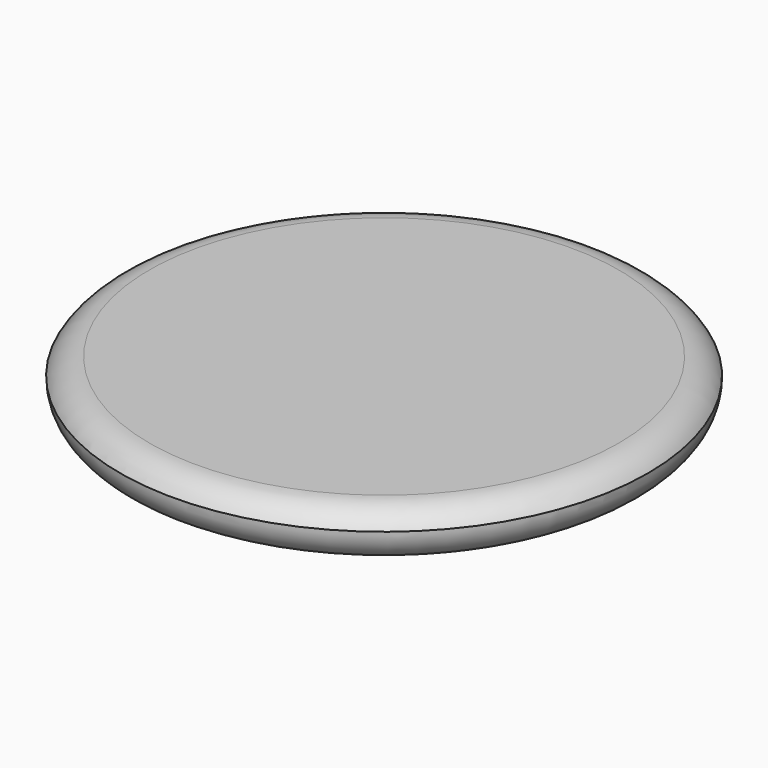
from build123d import *

# Parameters (mm, degrees)
F0_R     = 15.6
F0_R_2   = 5.6
F0_R_3   = 3.9
F1_DEPTH = 3
F2_DEPTH = 4
F3_DEPTH = 8
F4_R     = 2


# Not quite as in the source:
# - a fillet or chamfer that OpenCascade refuses, or shapes differently, is made with other operations: its cross-section is extruded or revolved along the edge and cut away or added


with BuildPart() as f1:
    # F0 (on Top) → F1 (new body)
    with BuildSketch(Plane.XY):
        Circle(F0_R)
        Circle(F0_R_2, mode=Mode.SUBTRACT)
        Circle(F0_R_2)
        Circle(F0_R_3, mode=Mode.SUBTRACT)
        Circle(F0_R_3)
    extrude(amount=-F1_DEPTH)

    # F0 (on Top) → F2 (join)
    with BuildSketch(Plane.XY):
        Circle(F0_R_2)
        Circle(F0_R_3, mode=Mode.SUBTRACT)
        Circle(F0_R_3)
    extrude(amount=-F2_DEPTH)

    # F0 (on Top) → F3 (join)
    with BuildSketch(Plane.XY):
        Circle(F0_R_3)
    extrude(amount=-F3_DEPTH)

    # F4
    f4_edges = [f1.edges().sort_by_distance(p)[0] for p in [
        (-15.6, 0, -3),
    ]]
    fillet(f4_edges, radius=F4_R)

    # F5: fillet of radius 2 on 1 edges, made by hand

    # F5_s1 → F5_t2 (revolve, cut)
    with BuildSketch(Plane.XZ):
        with BuildLine():
            ThreePointArc((15.6, -1), (14.8679491924, -0.2679491924), (13.8679491924, 0))
            Line((13.8679491924, 0), (15.6, 0))
            Line((15.6, 0), (15.6, -1))
        make_face()
    revolve(axis=Axis((0, 0, 0), (0, 0, 1)), mode=Mode.SUBTRACT)


solid = f1.part
